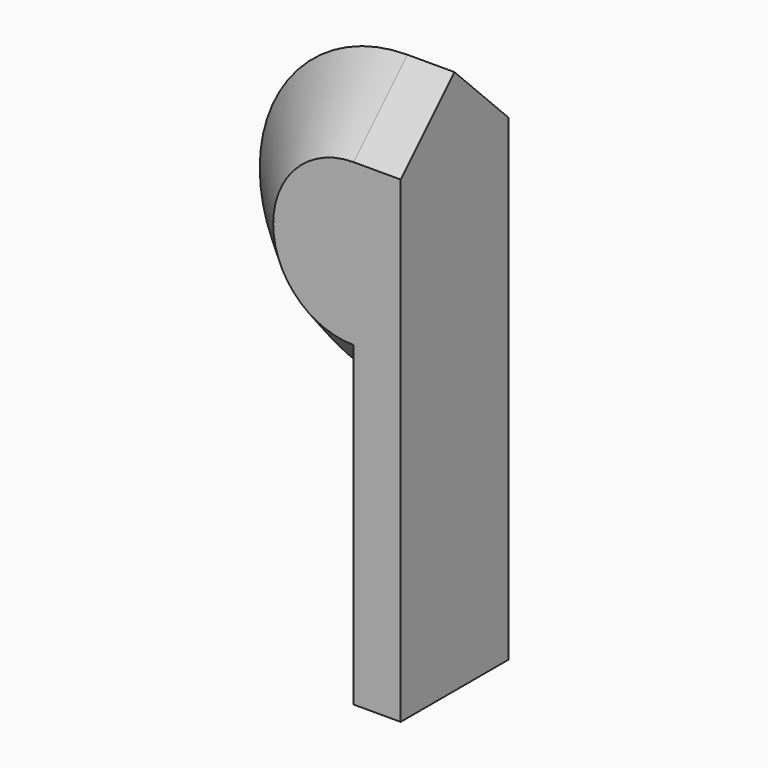
from build123d import *

# Parameters (mm, degrees)
F1_DEPTH = 25.4
F2_SIZE  = 12.69999


# Not quite as in the source:
# - a fillet or chamfer is up to 0.001 mm smaller than in the source, because OpenCascade refuses the exact size


with BuildPart() as f1:
    # F0 (on Front) → F1 (new body)
    with BuildSketch(Plane.XZ):
        with BuildLine():
            Line((8.873289451, 55.7964481413), (0, 55.7964481413))
            ThreePointArc((0, 55.7964481413), (-27.8982240707, 27.8982240707), (0, 0))
            Line((0, 0), (0, -47.0735542476))
            Line((0, -47.0735542476), (8.873289451, -47.0735542476))
            Line((8.873289451, -47.0735542476), (8.873289451, 55.7964481413))
        make_face()
    extrude(amount=F1_DEPTH)

    # F2 (size 12.7 in the source; OpenCascade refuses exactly that, so slightly less here)
    f2_edges = [f1.edges().sort_by_distance(p)[0] for p in [
        (-27.898224, -25.4, 27.898224),
        (-27.898224, 0, 27.898224),
    ]]
    chamfer(f2_edges, length=F2_SIZE)


solid = f1.part
